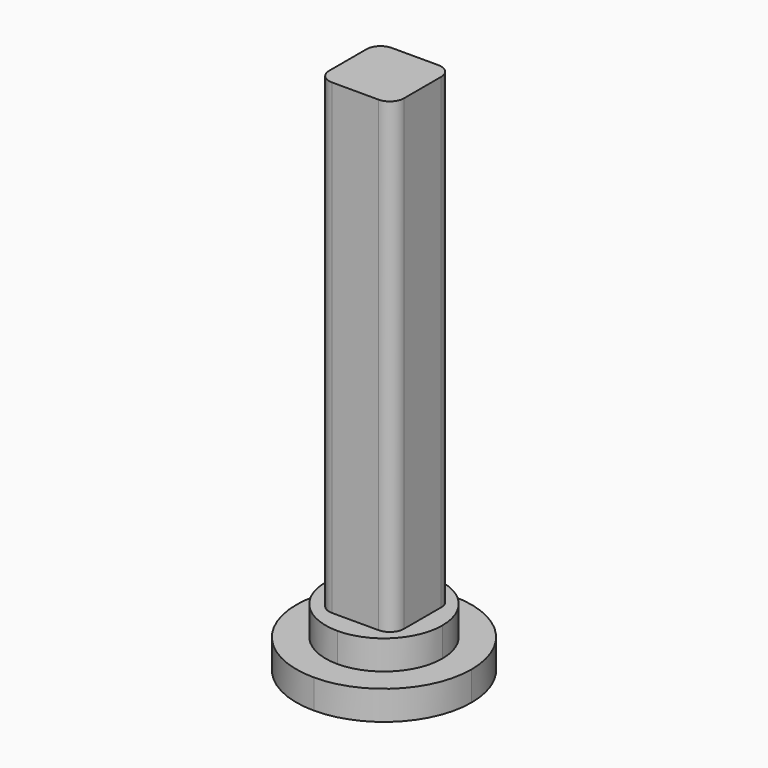
from build123d import *

# Parameters (mm, degrees)
F0_W     = 16.256
F0_H     = 16.256
F1_DEPTH = 114.3
F0_W_2   = 25.4
F0_H_2   = 25.4
F2_DEPTH = 12.7
F3_R     = 3.048
F4_R     = 12.69999
F0_W_3   = 38.1
F0_H_3   = 38.1
F5_DEPTH = 6.35
F6_R     = 19.04999


# Not quite as in the source:
# - a fillet or chamfer is up to 0.001 mm smaller than in the source, because OpenCascade refuses the exact size


with BuildPart() as f1:
    # F0 (on Top) → F1 (new body)
    with BuildSketch(Plane.XY):
        with Locations((8.128, 8.128)):
            Rectangle(F0_W, F0_H)
    extrude(amount=F1_DEPTH)

    # F0 (on Top) → F2 (join)
    with BuildSketch(Plane.XY):
        with Locations((7.8703831056, 8.128)):
            Rectangle(F0_W_2, F0_H_2)
        with Locations((8.128, 8.128)):
            Rectangle(F0_W, F0_H, mode=Mode.SUBTRACT)
    extrude(amount=F2_DEPTH)

    # F3
    f3_edges = [f1.edges().sort_by_distance(p)[0] for p in [
        (0, 16.256, 63.5),
        (16.256, 16.256, 63.5),
        (16.256, 0, 63.5),
        (0, 0, 63.5),
    ]]
    fillet(f3_edges, radius=F3_R)

    # F4 (radius 12.7 in the source; OpenCascade refuses exactly that, so slightly less here)
    f4_edges = [f1.edges().sort_by_distance(p)[0] for p in [
        (-4.829617, 20.828, 6.35),
        (-4.829617, -4.572, 6.35),
        (20.570383, -4.572, 6.35),
        (20.570383, 20.828, 6.35),
    ]]
    fillet(f4_edges, radius=F4_R)

    # F0 (on Top) → F5 (join)
    with BuildSketch(Plane.XY):
        with Locations((7.8703831056, 8.128)):
            Rectangle(F0_W_3, F0_H_3)
        with Locations((7.8703831056, 8.128)):
            Rectangle(F0_W_2, F0_H_2, mode=Mode.SUBTRACT)
        with Locations((7.8703831056, 8.128)):
            Rectangle(F0_W_2, F0_H_2)
        with Locations((8.128, 8.128)):
            Rectangle(F0_W, F0_H, mode=Mode.SUBTRACT)
    extrude(amount=F5_DEPTH)

    # F6 (radius 19.05 in the source; OpenCascade refuses exactly that, so slightly less here)
    f6_edges = [f1.edges().sort_by_distance(p)[0] for p in [
        (-11.179617, 27.178, 3.175),
        (26.920383, 27.178, 3.175),
        (26.920383, -10.922, 3.175),
        (-11.179617, -10.922, 3.175),
    ]]
    fillet(f6_edges, radius=F6_R)


solid = f1.part
